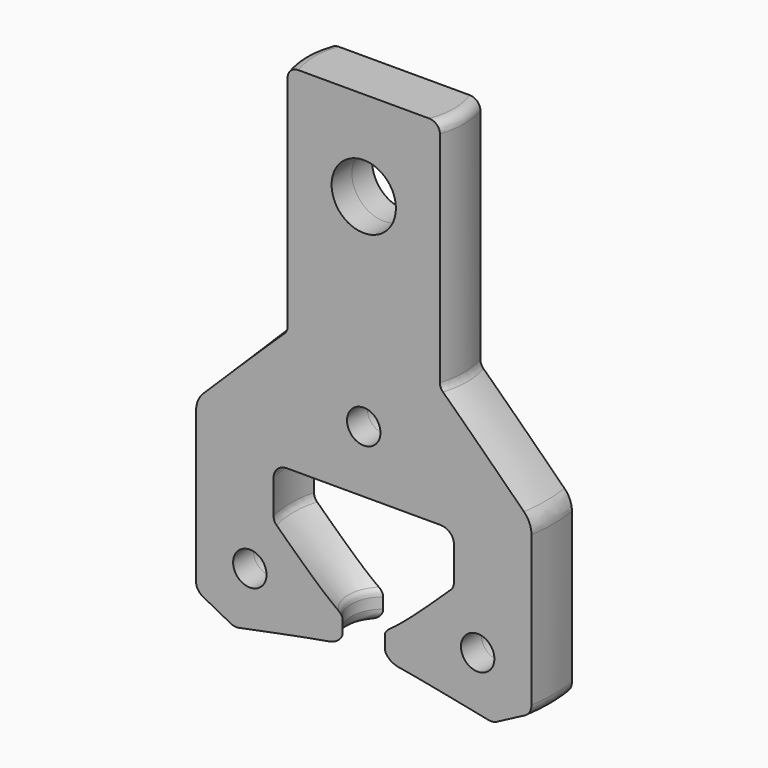
from build123d import *

# Parameters (mm, degrees)
F3_DEPTH      = 100.9656034356
F4_R          = 2
F5_R          = 6.35
F5_R_2        = 3.3
F6_DEPTH      = 5.0010027607
F6_DEPTH_BACK = 5.0010027607
F7_R          = 5
F8_R          = 2.5


# Not quite as in the source:
# - a feature names something its author has since deleted; it is built from what else it names


with BuildPart() as f1:
    # F0 (on Front) → F1 (revolve)
    with BuildSketch(Plane.XZ):
        with BuildLine():
            Line((0, 80.5346034356), (0, 67.8346034356))
            ThreePointArc((0, 67.8346034356), (4.4901280605, 69.6944753751), (6.35, 74.1846034356))
            ThreePointArc((6.35, 74.1846034356), (4.4901280605, 78.6747314961), (0, 80.5346034356))
        make_face()
        Polygon((18.5, 22), (18.5, 12), (18.5, 0), (33.5, 0), (33.5, 22), align=None)
        Polygon((18.5, 12), (6.5, 0), (18.5, 0), align=None)
        Polygon((18.5, 0), (6.5, 0), (6.5, -5), (33.5, -5), (33.5, 0), align=None)
        Polygon((33.5, -5), (6.5, -5), (26, -9), align=None)
        with BuildLine():
            Line((0, 22), (18.5, 22))
            Line((18.5, 22), (33.5, 22))
            Line((33.5, 22), (33.5, 28.2132034356))
            Line((33.5, 28.2132034356), (15.8496, 45.8636034356))
            Line((15.8496, 45.8636034356), (15.8496, 91.9646034356))
            Line((15.8496, 91.9646034356), (0, 91.9646034356))
            Line((0, 91.9646034356), (0, 80.5346034356))
            ThreePointArc((0, 80.5346034356), (4.4901280605, 78.6747314961), (6.35, 74.1846034356))
            ThreePointArc((6.35, 74.1846034356), (4.4901280605, 69.6944753751), (0, 67.8346034356))
            Line((0, 67.8346034356), (0, 22))
        make_face()
    revolve(axis=Axis((0, 0, 56.9823017178), (0, 0, -1)))

    # F2 (on face) → F3 (cut, through all)
    with BuildSketch(Plane.XY.offset(91.9646034356)):
        with BuildLine():
            ThreePointArc((15.0402732741, -5), (0, -15.8496), (-15.0402732741, -5))
            Line((-15.0402732741, -5), (-33.5, -5))
            Line((-33.5, -5), (-33.5, -33.5))
            Line((-33.5, -33.5), (33.5, -33.5))
            Line((33.5, -33.5), (33.5, -5))
            Line((33.5, -5), (15.0402732741, -5))
        make_face()
        with BuildLine():
            Line((33.5, 33.5), (-33.5, 33.5))
            Line((-33.5, 33.5), (-33.5, 5))
            Line((-33.5, 5), (-15.0402732741, 5))
            ThreePointArc((-15.0402732741, 5), (0, 15.8496), (15.0402732741, 5))
            Line((15.0402732741, 5), (33.5, 5))
            Line((33.5, 5), (33.5, 33.5))
        make_face()
        with BuildLine():
            Line((15.0402732741, -5), (-15.0402732741, -5))
            ThreePointArc((-15.0402732741, -5), (0, -15.8496), (15.0402732741, -5))
        make_face()
        with BuildLine():
            ThreePointArc((15.0402732741, 5), (0, 15.8496), (-15.0402732741, 5))
            Line((-15.0402732741, 5), (15.0402732741, 5))
        make_face()
    extrude(amount=-F3_DEPTH, mode=Mode.SUBTRACT)

    # F4
    f4_edges = [f1.edges().sort_by_distance(p)[0] for p in [
        (-15.8496, 0, 91.964603),
        (15.8496, 0, 91.964603),
        (-18.5, 0, 12),
        (18.5, 0, 12),
        (-15.8496, 0, 45.863603),
        (15.8496, 0, 45.863603),
        (-6.5, 0, 0),
        (6.5, 0, 0),
    ]]
    fillet(f4_edges, radius=F4_R)

    # F5 (on Front) → F6 (cut, two sides)
    with BuildSketch(Plane.XZ) as f6_sk:
        with Locations((0, 74.1846034356)):
            Circle(F5_R)
        with Locations((22.5, 2.1846034356)):
            Circle(F5_R_2)
        with Locations((0, 34.1846034356)):
            Circle(F5_R_2)
        with Locations((-22.5, 2.1846034356)):
            Circle(F5_R_2)
    extrude(amount=-F6_DEPTH, mode=Mode.SUBTRACT)
    extrude(f6_sk.sketch, amount=F6_DEPTH_BACK, mode=Mode.SUBTRACT)

    # F7
    f7_edges = [f1.edges().sort_by_distance(p)[0] for p in [
        (33.5, 0, 28.213203),
        (-33.5, 0, 28.213203),
    ]]
    fillet(f7_edges, radius=F7_R)

    # F8
    f8_edges = [f1.edges().sort_by_distance(p)[0] for p in [
        (-6.5, 0, -5),
        (6.5, 0, -5),
        (-26, 0, -9),
        (26, 0, -9),
        (33.5, 0, -5),
        (18.5, 0, 22),
        (-18.5, 0, 22),
        (-33.5, 0, -5),
    ]]
    fillet(f8_edges, radius=F8_R)


solid = f1.part
